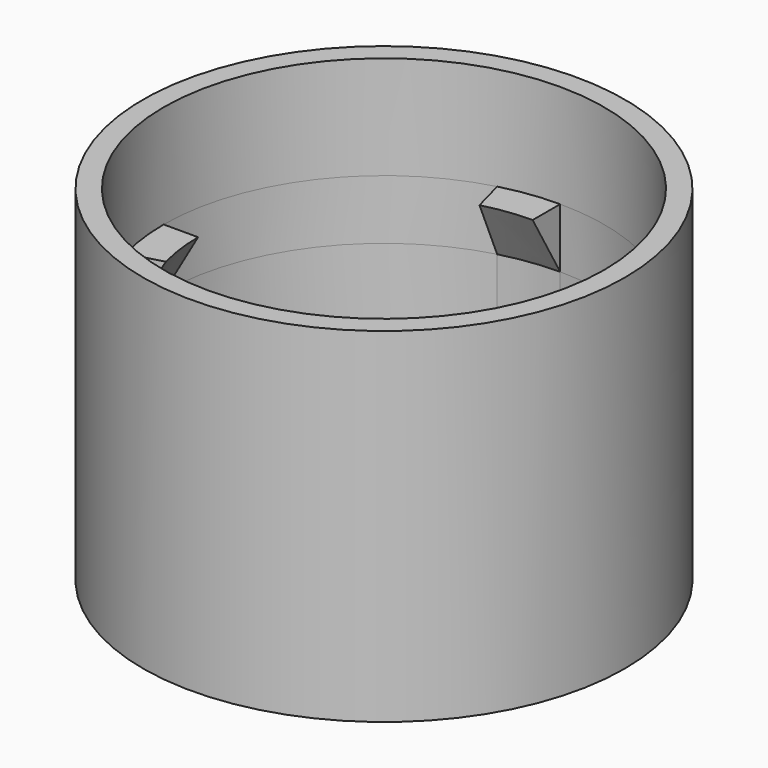
from build123d import *
from build123d import SkipClean  # not in build123d's __all__

# Parameters (mm, degrees)
F0_R     = 35
F1_DEPTH = 50
F2_T     = -3
F6_DEPTH = 25
F7_R     = 5
F8_DEPTH = 25


# Not quite as in the source:
# - after a boolean that leaves OpenCascade's solid faulty, fix() repairs it


with BuildPart() as f1:
    # F0 (on Top) → F1 (new body)
    with BuildSketch(Plane.XY):
        Circle(F0_R)
    extrude(amount=F1_DEPTH)

    # F2
    f2_openings = [f1.faces().sort_by_distance(p)[0] for p in [
        (0, 0, 50),
    ]]
    offset(amount=F2_T, openings=f2_openings)

    # F3 (on Right) → F4 (revolve)
    with BuildSketch(Plane.YZ):
        Polygon((-27, 35), (-32, 35), (-32, 26.3397459622), align=None)
    revolve(axis=Axis((0, 0, 50.3253415227), (0, 0, 1)))

    # F5 (on face) → F6 (cut)
    with BuildSketch(Plane.XY.offset(35)):
        with BuildLine():
            ThreePointArc((-8.2822094433, 30.9096264413), (-25.3873068893, 19.4803657283), (-32, 0))
            Line((-32, 0), (0, 0))
            Line((0, 0), (-8.2822094433, 30.9096264413))
        make_face()
        with BuildLine():
            Line((0, 32), (0, 0))
            Line((0, 0), (30.9096264413, 8.2822094433))
            ThreePointArc((30.9096264413, 8.2822094433), (19.4803657283, 25.3873068893), (0, 32))
        make_face()
        with BuildLine():
            Line((32, 0), (0, 0))
            Line((0, 0), (8.2822094433, -30.9096264413))
            ThreePointArc((8.2822094433, -30.9096264413), (25.3873068893, -19.4803657283), (32, 0))
        make_face()
        with BuildLine():
            Line((0, -32), (0, 0))
            Line((0, 0), (-30.9096264413, -8.2822094433))
            ThreePointArc((-30.9096264413, -8.2822094433), (-19.4803657283, -25.3873068893), (0, -32))
        make_face()
    with SkipClean():  # cleaning this boolean's faces spoils the solid; the shape is the same uncleaned
        extrude(amount=-F6_DEPTH, mode=Mode.SUBTRACT)

    # F7 (on face) → F8 (cut)
    with BuildSketch(Plane.XY.offset(3)):
        Circle(F7_R)
    extrude(amount=-F8_DEPTH, mode=Mode.SUBTRACT)

    add(f1.part.fix(), mode=Mode.REPLACE)


solid = f1.part
